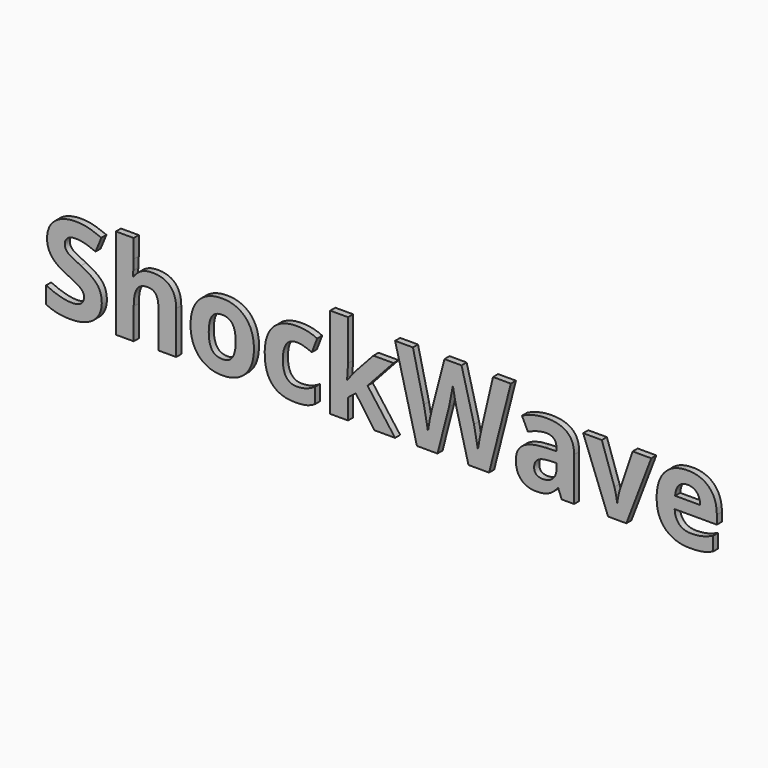
from build123d import *

# Parameters (mm, degrees)
F0_TEXT_SIZE = 188.1340725554
F1_DEPTH     = 10


# Not quite as in the source:
# - Text() gives the source's letters only with a copy of the font that has no kerning and outlines rounded to 1/6400 em; it was checked with that copy


with BuildPart() as f1:
    # F0 (on Front) → F1 (new body)
    with BuildSketch(Plane.XZ):
        with Locations((-501.8735546619, -58.5409402847)):
            Text('ShockWave', F0_TEXT_SIZE, font='Open Sans', font_style=FontStyle.BOLD, text_align=(TextAlign.LEFT, TextAlign.BOTTOM))
    extrude(amount=F1_DEPTH)


solid = f1.part
